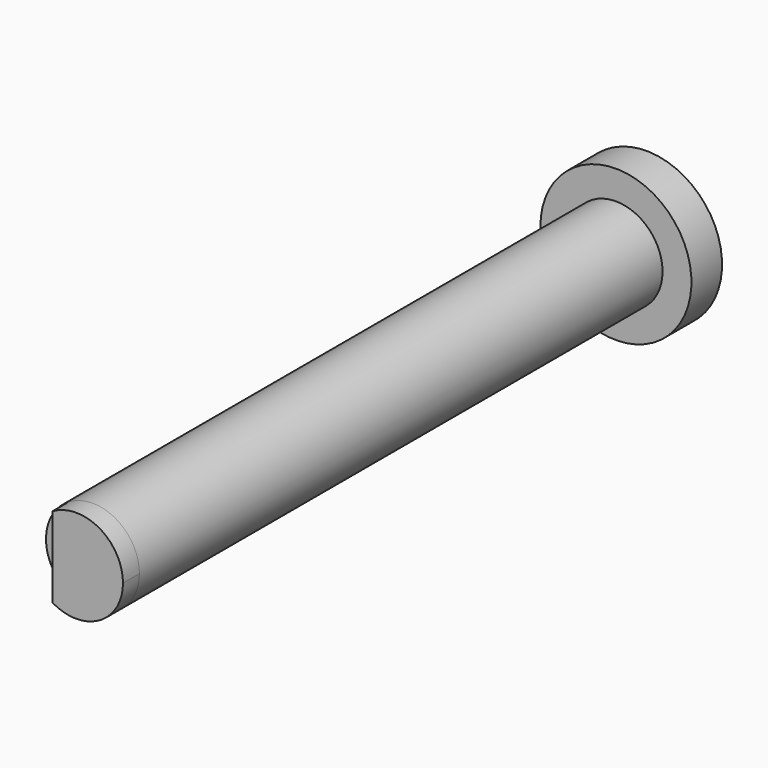
from build123d import *

# Parameters (mm, degrees)
F0_R     = 1.27
F1_DEPTH = 17.78
F2_R     = 2.0534537801
F3_DEPTH = 1.0414
F5_DEPTH = 0.5588


with BuildPart() as f1:
    # F0 (on Front) → F1 (new body)
    with BuildSketch(Plane.XZ):
        with Locations((-44.9135862291, 42.5175279379)):
            Circle(F0_R)
    extrude(amount=F1_DEPTH)

    # F2 (on face) → F3 (join)
    with BuildSketch(Plane(origin=(0, 0, 0), x_dir=(-1, 0, 0), z_dir=(0, 1, 0))):
        with Locations((44.9116155505, 42.5175279379)):
            Circle(F2_R)
        with BuildLine():
            ThreePointArc((44.2763268948, 41.4189832001), (43.6435862291, 42.5175279379), (44.2763268948, 43.6160726756))
            ThreePointArc((44.2763268948, 43.6160726756), (44.9113103393, 43.7875258986), (45.5469042063, 43.6183496036))
            ThreePointArc((45.5469042063, 43.6183496036), (46.0129528265, 43.1533683931), (46.1835862291, 42.5175279379))
            ThreePointArc((46.1835862291, 42.5175279379), (45.5474555553, 41.4170236547), (44.2763268948, 41.4189832001))
        make_face(mode=Mode.SUBTRACT)
        Polygon((44.2763268948, 43.6160726756), (44.2763268948, 42.5175279379), (44.2763268948, 41.4189832001), (45.5469042063, 41.4189832001), (45.5469042063, 43.6183496036), align=None)
        with BuildLine():
            Line((45.5469042063, 41.4189832001), (44.2763268948, 41.4189832001))
            ThreePointArc((44.2763268948, 41.4189832001), (45.5474555553, 41.4170236547), (46.1835862291, 42.5175279379))
            ThreePointArc((46.1835862291, 42.5175279379), (46.0129528265, 43.1533683931), (45.5469042063, 43.6183496036))
            Line((45.5469042063, 43.6183496036), (45.5469042063, 41.4189832001))
        make_face()
        with BuildLine():
            Line((44.2763268948, 41.4189832001), (44.2763268948, 42.5175279379))
            Line((44.2763268948, 42.5175279379), (44.2763268948, 43.6160726756))
            ThreePointArc((44.2763268948, 43.6160726756), (43.6435862291, 42.5175279379), (44.2763268948, 41.4189832001))
        make_face()
        with BuildLine():
            ThreePointArc((45.5469042063, 43.6183496036), (44.9113103393, 43.7875258986), (44.2763268948, 43.6160726756))
            Line((44.2763268948, 43.6160726756), (45.5469042063, 43.6183496036))
        make_face()
    extrude(amount=F3_DEPTH)

    # F4 (on face) → F5 (join)
    with BuildSketch(Plane.XZ.offset(17.78)):
        with BuildLine():
            Line((-45.5651804805, 43.6076311126), (-45.5651804805, 42.5175279379))
            Line((-45.5651804805, 42.5175279379), (-45.5651804805, 41.4274247632))
            ThreePointArc((-45.5651804805, 41.4274247632), (-44.2869382814, 41.4128957142), (-43.6435862291, 42.5175279379))
            ThreePointArc((-43.6435862291, 42.5175279379), (-44.2869382814, 43.6221601616), (-45.5651804805, 43.6076311126))
        make_face()
    extrude(amount=F5_DEPTH)


solid = f1.part
